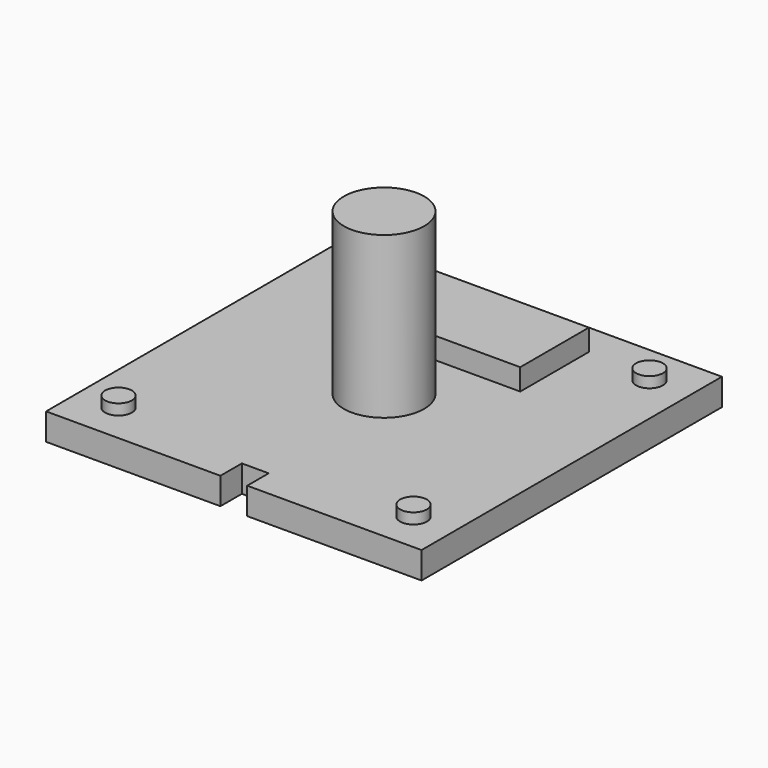
from build123d import *

# Parameters (mm, degrees)
F0_W            = 88.9
F0_H            = 88.9
F1_DEPTH        = 6.35
F2_R            = 9.525
F3_DEPTH        = 38.1
F4_W            = 38.1
F4_H            = 20.32
F5_DEPTH        = 5.08
F6_R            = 3.175
F7_DEPTH        = 10.16
F7_DEPTH_BACK   = 2.54
F7_COPIES_COUNT = 4
F8_W            = 6.35
F8_H            = 6.35
F9_DEPTH        = 6.35


# Not quite as in the source:
# - a pattern or mirror of a feature is missing from the dataset's text; its kind, count and spacing are read off the source's solid


with BuildPart() as f1:
    # F0 (on Top) → F1 (new body)
    with BuildSketch(Plane.XY):
        Rectangle(F0_W, F0_H)
    extrude(amount=F1_DEPTH)

    # F2 (on face) → F3 (join)
    with BuildSketch(Plane.XY.offset(6.35)):
        Circle(F2_R)
    extrude(amount=F3_DEPTH)

    # F4 (on face) → F5 (join)
    with BuildSketch(Plane.XY.offset(6.35)):
        with Locations((0, 26.67)):
            Rectangle(F4_W, F4_H)
    extrude(amount=F5_DEPTH)

    # F6 (on face) → F7 (join, two sides)
    with BuildSketch(Plane.XY.offset(6.35)) as f7_sk:
        with Locations((-34.925, 34.925)):
            Circle(F6_R)
    f7 = extrude(amount=-F7_DEPTH) + extrude(f7_sk.sketch, amount=F7_DEPTH_BACK)

    # F7_copies: F7 ×4 about axis
    f7_copies_axis = Axis((0, 0, 0), (0, 0, 1))
    for i in range(1, F7_COPIES_COUNT):
        add(f7.rotate(f7_copies_axis, i * 360 / F7_COPIES_COUNT))

    # F8 (on face) → F9 (cut)
    with BuildSketch(Plane.XY.offset(6.35)):
        with Locations((0, -41.275)):
            Rectangle(F8_W, F8_H)
    extrude(amount=-F9_DEPTH, mode=Mode.SUBTRACT)


solid = f1.part
